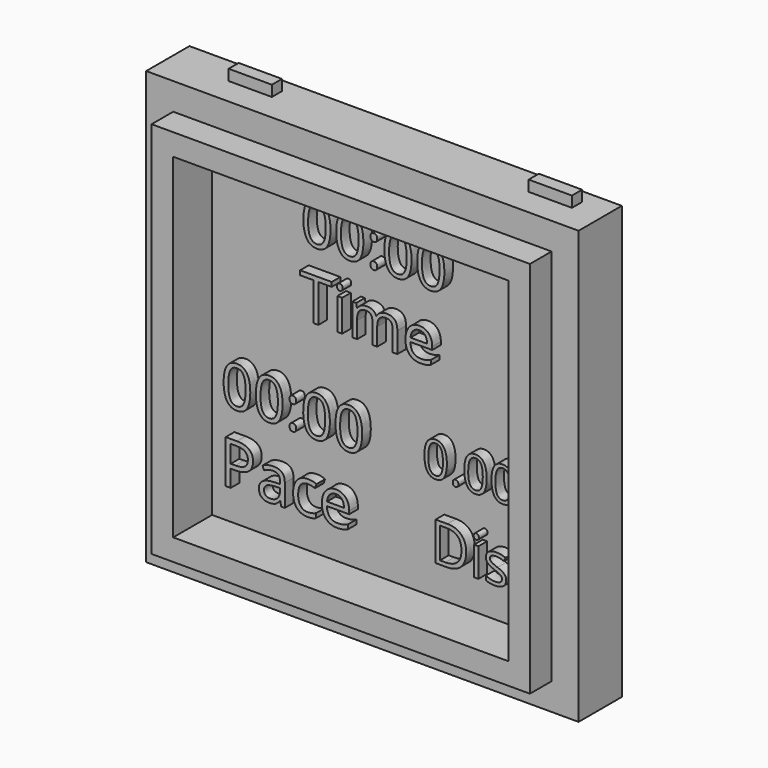
from build123d import *

# Parameters (mm, degrees)
F0_W           = 50.8
F0_H           = 50.8
F1_DEPTH       = 3.175
F2_W           = 44.45
F2_H           = 44.45
F3_DEPTH       = 3.175
F4_T           = -2.54
F5_TEXT_SIZE   = 6.7510577436
F5_TEXT_SIZE_2 = 6.9396754649
F5_TEXT_SIZE_3 = 6.6335714008
F5_TEXT_SIZE_4 = 7.0947261217
F5_TEXT_SIZE_5 = 5.5897816007
F5_TEXT_SIZE_6 = 6.3066849382
F8_DEPTH       = 1.27
F6_W           = 4.787709564
F6_H           = 1.5652128495
F6_W_2         = 5.08
F9_DEPTH       = 1.27
F7_W           = 5.08
F7_H           = 1.4959711116
F7_H_2         = 1.4830461005
F10_DEPTH      = 1.27


# Not quite as in the source:
# - Text() gives the source's letters only with a copy of the font that has no kerning and outlines rounded to 1/6400 em; it was checked with that copy


with BuildPart() as f1:
    # F0 (on Front) → F1 (new body, symmetric)
    with BuildSketch(Plane.XZ):
        Rectangle(F0_W, F0_H)
    extrude(amount=F1_DEPTH, both=True)

    # F2 (on face) → F3 (join, symmetric)
    with BuildSketch(Plane.XZ.offset(3.175)):
        Rectangle(F2_W, F2_H)
    extrude(amount=F3_DEPTH, both=True)

    # F4
    f4_openings = [f1.faces().sort_by_distance(p)[0] for p in [
        (0, -6.35, 0),
    ]]
    offset(amount=F4_T, openings=f4_openings, kind=Kind.INTERSECTION)

    # F5 (on face) → F8 (join, symmetric)
    with BuildSketch(Plane.XZ.offset(-0.635)):
        with Locations((-9.2999211047, 11.9181191549)):
            Text('00:00', F5_TEXT_SIZE, font='Open Sans', text_align=(TextAlign.LEFT, TextAlign.BOTTOM))
        with Locations((-9.4104763702, 4.024193855)):
            Text('Time', F5_TEXT_SIZE_2, font='Open Sans', text_align=(TextAlign.LEFT, TextAlign.BOTTOM))
        with Locations((-18.6648182571, -7.9053165391)):
            Text('00:00', F5_TEXT_SIZE_3, font='Open Sans', text_align=(TextAlign.LEFT, TextAlign.BOTTOM))
        with Locations((-18.7867712229, -16.1796100438)):
            Text('Pace', F5_TEXT_SIZE_4, font='Open Sans', text_align=(TextAlign.LEFT, TextAlign.BOTTOM))
        with Locations((4.9777391832, -7.4115763418)):
            Text('0.00', F5_TEXT_SIZE_5, font='Open Sans', text_align=(TextAlign.LEFT, TextAlign.BOTTOM))
        with Locations((5.9488911647, -16.1266587675)):
            Text('Dis', F5_TEXT_SIZE_6, font='Open Sans', text_align=(TextAlign.LEFT, TextAlign.BOTTOM))
    extrude(amount=F8_DEPTH, both=True)

    # F6 (on face) → F9 (join, symmetric)
    with BuildSketch(Plane(origin=(0, 0, -25.4), x_dir=(1, 0, 0), z_dir=(0, 0, -1))):
        with Locations((-19.8874119669, -0.7826064248)):
            Rectangle(F6_W, F6_H)
        with Locations((18.7445583129, -0.7826064248)):
            Rectangle(F6_W_2, F6_H)
    extrude(amount=F9_DEPTH, both=True)

    # F7 (on face) → F10 (join, symmetric)
    with BuildSketch(Plane.XY.offset(25.4)):
        with Locations((19.5394719326, 0.7479855558)):
            Rectangle(F7_W, F7_H)
        with Locations((-15.7134828782, 0.7415230502)):
            Rectangle(F7_W, F7_H_2)
    extrude(amount=F10_DEPTH, both=True)


solid = f1.part
